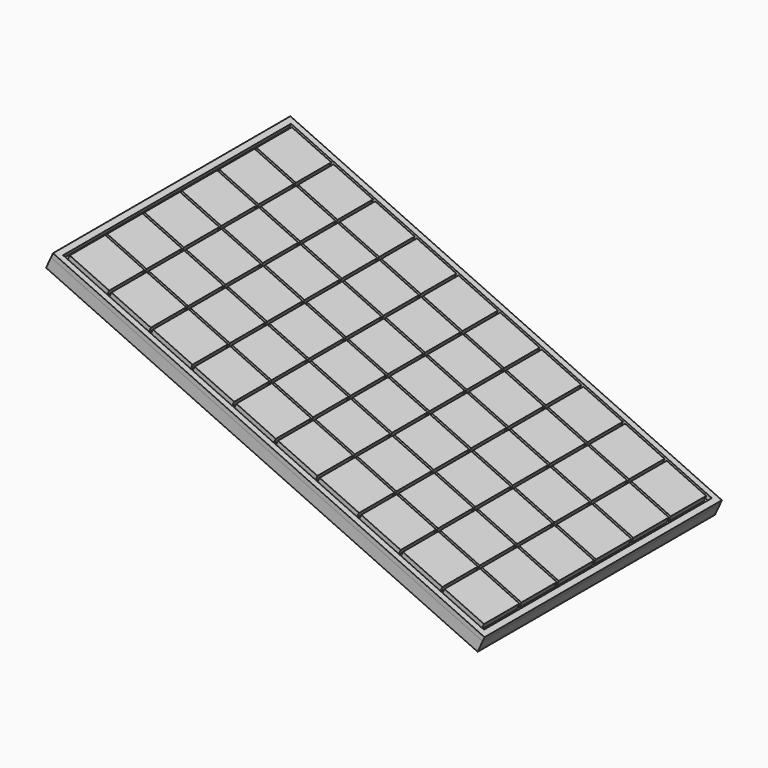
from build123d import *

# Parameters (mm, degrees)
F1_DEPTH = 1250
F2_W     = 183
F2_H     = 186.68
F2_H_2   = 186.66
F2_H_3   = 186.6600047684
F2_W_2   = 183.0000023842
F2_W_3   = 183.0000047684
F3_DEPTH = 25
F4_W     = 2000
F4_H     = 1250
F4_W_2   = 1950
F4_H_2   = 1200
F5_DEPTH = 20


# Not quite as in the source:
# - ends of sketch curves that miss each other by under 0.0002 mm in the source are joined


with BuildPart() as f1:
    # F0 (on Front) → F1 (new body)
    with BuildSketch(Plane.XZ):
        Polygon((-1818.2606033445, 833.0236361144), (0, 0), (20.8255909029, 45.4565150836), (-1797.4350124417, 878.480151198), align=None)
    extrude(amount=-F1_DEPTH)

    # F2 (on face) → F3 (join)
    with BuildSketch(Plane(origin=(20.8255909029, 0, 45.4565150836), x_dir=(0.9091303017, 0, -0.4165118181), z_dir=(0.4165118181, 0, 0.9091303017))):
        with Locations((-1868.5, 133.34)):
            Rectangle(F2_W, F2_H)
        with Locations((-1868.5, 330.01)):
            Rectangle(F2_W, F2_H_2)
        with Locations((-1868.5, 526.6700023842)):
            Rectangle(F2_W, F2_H_3)
        with Locations((-1868.5, 723.33)):
            Rectangle(F2_W, F2_H_2)
        with Locations((-1868.5, 919.99)):
            Rectangle(F2_W, F2_H_2)
        with Locations((-1868.5, 1116.66)):
            Rectangle(F2_W, F2_H)
        with Locations((-1675.5, 133.34)):
            Rectangle(F2_W, F2_H)
        with Locations((-1675.5, 330.01)):
            Rectangle(F2_W, F2_H_2)
        with Locations((-1675.5, 526.6700023842)):
            Rectangle(F2_W, F2_H_3)
        with Locations((-1675.5, 723.33)):
            Rectangle(F2_W, F2_H_2)
        with Locations((-1675.5, 919.99)):
            Rectangle(F2_W, F2_H_2)
        with Locations((-1675.5, 1116.66)):
            Rectangle(F2_W, F2_H)
        with Locations((-1482.5, 1116.66)):
            Rectangle(F2_W, F2_H)
        with Locations((-1482.5, 919.99)):
            Rectangle(F2_W, F2_H_2)
        with Locations((-1482.5, 723.33)):
            Rectangle(F2_W, F2_H_2)
        with Locations((-1482.5, 526.6700023842)):
            Rectangle(F2_W, F2_H_3)
        with Locations((-1482.5, 330.01)):
            Rectangle(F2_W, F2_H_2)
        with Locations((-1482.5, 133.34)):
            Rectangle(F2_W, F2_H)
        with Locations((-1289.5, 133.34)):
            Rectangle(F2_W, F2_H)
        with Locations((-1289.5, 330.01)):
            Rectangle(F2_W, F2_H_2)
        with Locations((-1289.5, 526.6700023842)):
            Rectangle(F2_W, F2_H_3)
        with Locations((-1289.5, 723.33)):
            Rectangle(F2_W, F2_H_2)
        with Locations((-1289.5, 919.99)):
            Rectangle(F2_W, F2_H_2)
        with Locations((-1289.5, 1116.66)):
            Rectangle(F2_W, F2_H)
        Polygon((-1004.9999976158, 226.68), (-1188, 226.68), (-1188, 40), (-1005, 40), align=None)
        with Locations((-1096.4999988079, 330.01)):
            Rectangle(F2_W_2, F2_H_2)
        with Locations((-1096.4999988079, 526.6700023842)):
            Rectangle(F2_W_2, F2_H_3)
        with Locations((-1096.4999988079, 723.33)):
            Rectangle(F2_W_2, F2_H_2)
        with Locations((-1096.4999988079, 919.99)):
            Rectangle(F2_W_2, F2_H_2)
        Polygon((-1005, 1210), (-1188, 1210), (-1188, 1023.32), (-1004.9999976158, 1023.32), align=None)
        Polygon((-812, 226.68), (-995.0000023842, 226.68), (-995.0000047684, 40), (-812, 40), align=None)
        Polygon((-812, 423.34), (-995.0000023842, 423.34), (-995.0000047684, 236.68), (-812, 236.68), align=None)
        Polygon((-812, 620.0000047684), (-995.0000023842, 620.0000047684), (-995.0000047684, 433.34), (-812, 433.34), align=None)
        Polygon((-812, 816.66), (-995.0000023842, 816.66), (-995.0000047684, 630), (-812, 630), align=None)
        Polygon((-812, 1013.32), (-995.0000023842, 1013.32), (-995.0000047684, 826.66), (-812, 826.66), align=None)
        with Locations((-903.5000023842, 1116.66)):
            Rectangle(F2_W_3, F2_H)
        with Locations((-710.5, 1116.66)):
            Rectangle(F2_W, F2_H)
        with Locations((-710.5, 919.99)):
            Rectangle(F2_W, F2_H_2)
        with Locations((-710.5, 723.33)):
            Rectangle(F2_W, F2_H_2)
        with Locations((-710.5, 526.6700023842)):
            Rectangle(F2_W, F2_H_3)
        with Locations((-710.5, 330.01)):
            Rectangle(F2_W, F2_H_2)
        with Locations((-710.5, 133.34)):
            Rectangle(F2_W, F2_H)
        with Locations((-517.5, 133.34)):
            Rectangle(F2_W, F2_H)
        with Locations((-517.5, 330.01)):
            Rectangle(F2_W, F2_H_2)
        with Locations((-517.5, 526.6700023842)):
            Rectangle(F2_W, F2_H_3)
        with Locations((-517.5, 723.33)):
            Rectangle(F2_W, F2_H_2)
        with Locations((-517.5, 919.99)):
            Rectangle(F2_W, F2_H_2)
        with Locations((-517.5, 1116.66)):
            Rectangle(F2_W, F2_H)
        with Locations((-324.5, 1116.66)):
            Rectangle(F2_W, F2_H)
        with Locations((-324.5, 919.99)):
            Rectangle(F2_W, F2_H_2)
        with Locations((-324.5, 723.33)):
            Rectangle(F2_W, F2_H_2)
        with Locations((-324.5, 526.6700023842)):
            Rectangle(F2_W, F2_H_3)
        with Locations((-324.5, 330.01)):
            Rectangle(F2_W, F2_H_2)
        with Locations((-324.5, 133.34)):
            Rectangle(F2_W, F2_H)
        with Locations((-131.5, 133.34)):
            Rectangle(F2_W, F2_H)
        with Locations((-131.5, 330.01)):
            Rectangle(F2_W, F2_H_2)
        with Locations((-131.5, 526.6700023842)):
            Rectangle(F2_W, F2_H_3)
        with Locations((-131.5, 723.33)):
            Rectangle(F2_W, F2_H_2)
        with Locations((-131.5, 919.99)):
            Rectangle(F2_W, F2_H_2)
        with Locations((-131.5, 1116.66)):
            Rectangle(F2_W, F2_H)
    extrude(amount=F3_DEPTH)


with BuildPart() as f5:
    # F4 (on face) → F5 (new body)
    with BuildSketch(Plane(origin=(20.8255909029, 0, 45.4565150836), x_dir=(0.9091303017, 0, -0.4165118181), z_dir=(0.4165118181, 0, 0.9091303017))):
        with Locations((-1000, 625)):
            Rectangle(F4_W, F4_H)
        with Locations((-1000, 625)):
            Rectangle(F4_W_2, F4_H_2, mode=Mode.SUBTRACT)
    extrude(amount=F5_DEPTH)


solid = Compound([f1.part, f5.part])
